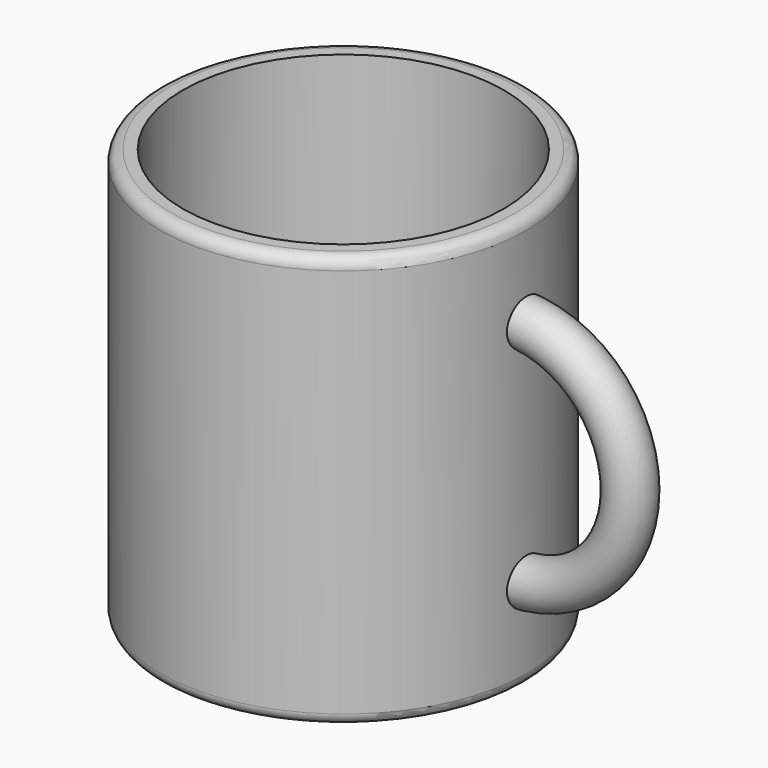
from build123d import *

# Parameters (mm, degrees)
F0_R         = 40
F1_DEPTH     = 90
F2_T         = -5
F4_R         = 5
F5_ANGLE     = 180
F6_R         = 2.5
F7_TEXT_SIZE = 32.762859741
F8_DEPTH     = 2.5


# Not quite as in the source:
# - Text() gives the source's letters only with a copy of the font that has no kerning and outlines rounded to 1/6400 em; it was checked with that copy


with BuildPart() as f1:
    # F0 (on Top) → F1 (new body)
    with BuildSketch(Plane.XY):
        Circle(F0_R)
    extrude(amount=F1_DEPTH)

    # F2
    f2_openings = [f1.faces().sort_by_distance(p)[0] for p in [
        (0, 0, 90),
    ]]
    offset(amount=F2_T, openings=f2_openings)

    # F6
    f6_edges = [f1.edges().sort_by_distance(p)[0] for p in [
        (-40, 0, 90),
        (-40, 0, 0),
    ]]
    fillet(f6_edges, radius=F6_R)

    # F7 (on face) → F8 (cut)
    with BuildSketch(Plane(origin=(0, 0, 0), x_dir=(1, 0, 0), z_dir=(0, 0, -1))):
        with Locations((-32.824290103, -12.509454973)):
            Text('Paul', F7_TEXT_SIZE, font='Open Sans', text_align=(TextAlign.LEFT, TextAlign.BOTTOM))
    extrude(amount=-F8_DEPTH, mode=Mode.SUBTRACT)


with BuildPart() as f5:
    # F4 (on offset) → F5 (revolve)
    with BuildSketch(Plane.YZ.offset(37.5)):
        with Locations((0, 70)):
            Circle(F4_R)
    revolve(axis=Axis((37.5, 13.7604000047, 45), (0, 1, 0)), revolution_arc=F5_ANGLE)


solid = Compound([f1.part, f5.part])
